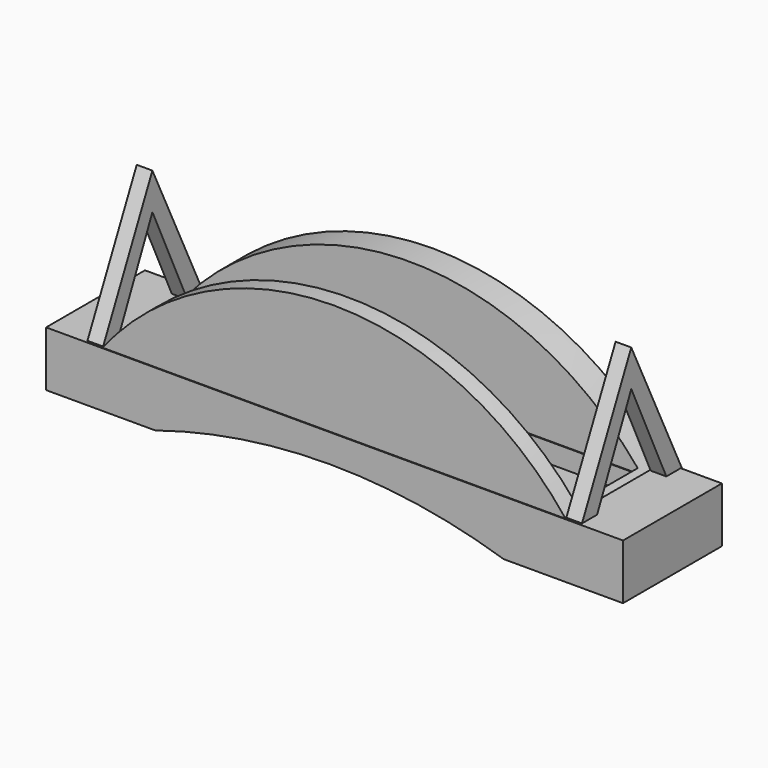
from build123d import *

# Parameters (mm, degrees)
F0_W      = 177.8
F0_H      = 38.1
F1_DEPTH  = 5.588
F4_DEPTH  = 4.826
F6_DEPTH  = 11.43
F8_DEPTH  = 233.426
F11_DEPTH = 38.1
F13_W     = 139.2178796232
F13_H     = 23.7698024139
F14_DEPTH = 51.308


with BuildPart() as f1:
    # F0 (on Top) → F1 (new body)
    with BuildSketch(Plane.XY):
        Rectangle(F0_W, F0_H)
    extrude(amount=F1_DEPTH)

    # F3 (on offset) → F4 (join)
    with BuildSketch(Plane.YZ.offset(76.2)):
        Polygon((0, 46.0882298648), (-18.9831927419, 6.0590645298), (-13.1481755525, 6.0590645298), (0, 34.8115004599), (13.6455185711, 5.3136325441), (19.5630453527, 5.3136325441), align=None)
    extrude(amount=-F4_DEPTH)

    # F5: F1 across plane


with BuildPart() as f1_1:
    add(f1.part)
    add(f1.part.mirror(Plane.YZ))

    # F6 (add): a face of the model
    f6_faces = [f1_1.faces().sort_by_distance(p)[0] for p in [
        (0, 0, 0),
    ]]
    extrude(f6_faces, amount=F6_DEPTH)

    # F7 (on face) → F8 (cut)
    with BuildSketch(Plane.XZ.offset(19.05)):
        with BuildLine():
            Line((-55.2403405309, -11.43), (52.1429181099, -11.43))
            ThreePointArc((52.1429181099, -11.43), (-1.5487112105, -3.1079738738), (-55.2403405309, -11.43))
        make_face()
    extrude(amount=-F8_DEPTH, mode=Mode.SUBTRACT)

    # F10 (on offset) → F11 (join)
    with BuildSketch(Plane.XZ.offset(19.05)):
        with BuildLine():
            Line((-71.5217785408, 5.7395980693), (71.2262214592, 5.7395980693))
            ThreePointArc((71.2262214592, 5.7395980693), (-0.1477785408, 40.3939508929), (-71.5217785408, 5.7395980693))
        make_face()
    extrude(amount=-F11_DEPTH)

    # F13 (on offset) → F14 (cut)
    with BuildSketch(Plane.XY.offset(50.8254)):
        with Locations((0.4383567721, -1.7096721567)):
            Rectangle(F13_W, F13_H)
    extrude(amount=-F14_DEPTH, mode=Mode.SUBTRACT)


solid = f1_1.part
